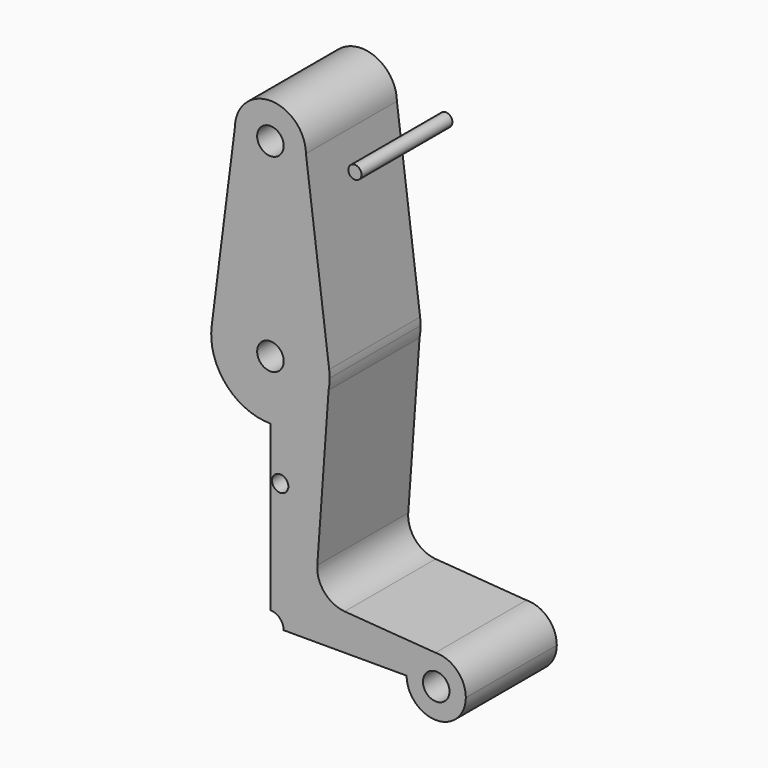
from build123d import *

# Parameters (mm, degrees)
F0_R     = 2.1842909743
F1_DEPTH = 30.48
F0_R_2   = 1.7632939696


with BuildPart() as f1:
    # F0 (on Front) → F1 (new body)
    with BuildSketch(Plane.XZ):
        with BuildLine():
            ThreePointArc((-9.5243800429, 114.4086728964), (-6.7735047921, 107.6033398002), (0, 104.775))
            ThreePointArc((0, 104.775), (6.7351920908, 107.5648079092), (9.525, 114.3))
            ThreePointArc((9.525, 114.3), (9.5248450095, 114.3543373324), (9.5243800429, 114.4086728964))
            ThreePointArc((9.5243800429, 114.4086728964), (0, 123.825), (-9.5243800429, 114.4086728964))
        make_face()
        with BuildLine():
            ThreePointArc((3.556, 114.3), (2.5144717139, 111.7855282861), (0, 110.744))
            ThreePointArc((0, 110.744), (-2.5144717139, 116.8144717139), (3.556, 114.3))
        make_face(mode=Mode.SUBTRACT)
        with BuildLine():
            ThreePointArc((9.525, 114.3), (6.7351920908, 107.5648079092), (0, 104.775))
            Line((0, 104.775), (0, 79.375))
            ThreePointArc((0, 79.375), (10.4928697542, 75.4128212159), (15.7479913604, 65.5040940878))
            Line((15.7479913604, 65.5040940878), (9.5243800429, 114.4086728964))
            ThreePointArc((9.5243800429, 114.4086728964), (9.5248450095, 114.3543373324), (9.525, 114.3))
        make_face()
        with BuildLine():
            Line((0, 79.375), (0, 104.775))
            ThreePointArc((0, 104.775), (-6.7735047921, 107.6033398002), (-9.5243800429, 114.4086728964))
            Line((-9.5243800429, 114.4086728964), (-15.7479913604, 65.5040940878))
            ThreePointArc((-15.7479913604, 65.5040940878), (-10.4928697542, 75.4128212159), (0, 79.375))
        make_face()
        with BuildLine():
            ThreePointArc((15.7479913604, 65.5040940878), (10.4928697542, 75.4128212159), (0, 79.375))
            Line((0, 79.375), (0, 67.056))
            ThreePointArc((0, 67.056), (2.5144717139, 66.0144717139), (3.556, 63.5))
            ThreePointArc((3.556, 63.5), (2.5144717139, 60.9855282861), (0, 59.944))
            Line((0, 59.944), (0, 47.625))
            ThreePointArc((0, 47.625), (10.1293130273, 51.2765535713), (15.5987546644, 60.5513599881))
            ThreePointArc((15.5987546644, 60.5513599881), (15.8057877896, 62.0192240712), (15.875, 63.5))
            ThreePointArc((15.875, 63.5), (15.8432160221, 64.5040573076), (15.7479913604, 65.5040940878))
        make_face()
        with BuildLine():
            Line((0, 67.056), (0, 79.375))
            ThreePointArc((0, 79.375), (-10.4928697542, 75.4128212159), (-15.7479913604, 65.5040940878))
            ThreePointArc((-15.7479913604, 65.5040940878), (-15.8677980625, 63.0218685866), (-15.5987546644, 60.5513599881))
            ThreePointArc((-15.5987546644, 60.5513599881), (-10.1293130273, 51.2765535713), (0, 47.625))
            Line((0, 47.625), (0, 59.944))
            ThreePointArc((0, 59.944), (-3.556, 63.5), (0, 67.056))
        make_face()
        with BuildLine():
            ThreePointArc((15.5987546644, 60.5513599881), (10.1293130273, 51.2765535713), (0, 47.625))
            Line((0, 47.625), (0, 11.2290981952))
            ThreePointArc((0, 11.2290981952), (7.9401714804, 7.9401714804), (11.2290981952, 0))
            Line((11.2290981952, 0), (36.5125, 0))
            ThreePointArc((36.5125, 0), (38.764717935, 5.539086034), (44.2432651255, 7.9348073034))
            Line((44.2432651255, 7.9348073034), (19.9053036746, 9.7469774609))
            ThreePointArc((19.9053036746, 9.7469774609), (14.4792388722, 12.4782393627), (12.5657807814, 18.2437097642))
            Line((12.5657807814, 18.2437097642), (15.5987546644, 60.5513599881))
        make_face()
        with Locations((2.6209076754, 34.3253262466)):
            Circle(F0_R, mode=Mode.SUBTRACT)
        with BuildLine():
            ThreePointArc((11.2290981952, 0), (7.9401714804, 7.9401714804), (0, 11.2290981952))
            Line((0, 11.2290981952), (0, 3.556))
            ThreePointArc((0, 3.556), (2.5144717139, 2.5144717139), (3.556, 0))
            Line((3.556, 0), (11.2290981952, 0))
        make_face()
        with BuildLine():
            ThreePointArc((44.2432651255, 7.9348073034), (38.764717935, 5.539086034), (36.5125, 0))
            ThreePointArc((36.5125, 0), (44.45, -7.9375), (52.3875, 0))
            ThreePointArc((52.3875, 0), (49.989086034, 5.685282065), (44.2432651255, 7.9348073034))
        make_face()
        with BuildLine():
            ThreePointArc((48.006, 0), (44.45, -3.556), (40.894, 0))
            ThreePointArc((40.894, 0), (44.45, 3.556), (48.006, 0))
        make_face(mode=Mode.SUBTRACT)
    extrude(amount=F1_DEPTH)


with BuildPart() as f1b:
    # F0 (on Front) → F1, piece 2 (new body)
    with BuildSketch(Plane.XZ):
        with Locations((22.6452313364, 114.3)):
            Circle(F0_R_2)
    extrude(amount=F1_DEPTH)


solid = Compound([f1.part, f1b.part])
